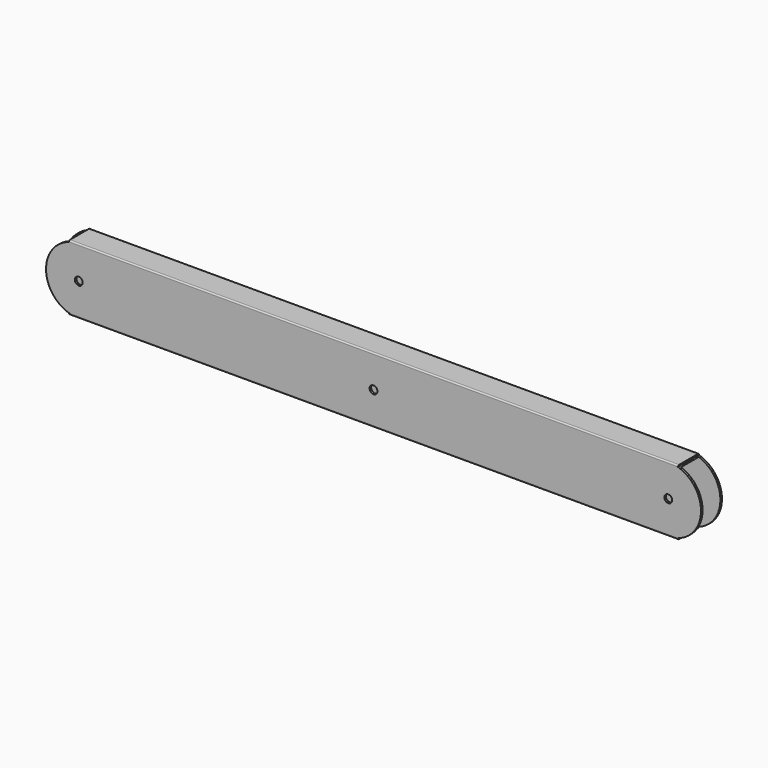
from build123d import *

# Parameters (mm, degrees)
F3_W     = 34
F3_H     = 94
F4_DEPTH = 500
F6_D     = 12
F6_DEPTH = 40
F6_TIP   = 3.6051637142
F7_DEPTH = 40
F8_DEPTH = 35
F9_DEPTH = 35


# Not quite as in the source:
# - a feature names something its author has since deleted; it is built from what else it names


with BuildPart() as f4:
    # F3 (on Right) → F4 (new body, symmetric)
    with BuildSketch(Plane.YZ):
        with BuildLine():
            ThreePointArc((-4.2945303673, -84.5), (-3.7087439297, -85.9142135624), (-2.2945303673, -86.5))
            Line((-2.2945303673, -86.5), (33.7054696327, -86.5))
            ThreePointArc((33.7054696327, -86.5), (35.1196831951, -85.9142135624), (35.7054696327, -84.5))
            Line((35.7054696327, -84.5), (35.7054696327, 11.5))
            ThreePointArc((35.7054696327, 11.5), (35.1196831951, 12.9142135624), (33.7054696327, 13.5))
            Line((33.7054696327, 13.5), (-2.2945303673, 13.5))
            ThreePointArc((-2.2945303673, 13.5), (-3.7087439297, 12.9142135624), (-4.2945303673, 11.5))
            Line((-4.2945303673, 11.5), (-4.2945303673, -84.5))
        make_face()
        with Locations((15.7054696327, -36.5)):
            Rectangle(F3_W, F3_H, mode=Mode.SUBTRACT)
    extrude(amount=F4_DEPTH, both=True)

    # F6
    with Locations(Plane.XZ.offset(4.2945303673)):
        with Locations((450, -36.2195856869), (0, -36.2195856869), (-450, -36.5)):
            Hole(F6_D / 2, depth=F6_DEPTH)
            with Locations((0, 0, -(F6_DEPTH + F6_TIP / 2))):  # 118° drill point
                Cone(0, F6_D / 2, F6_TIP, mode=Mode.SUBTRACT)

    # F5 (on face) → F7 (cut)
    with BuildSketch(Plane.XZ.offset(4.2945303673)):
        with BuildLine():
            ThreePointArc((-500, -36.5), (-490, -6.5), (-464, 11.5))
            Line((-464, 11.5), (-500, 11.5))
            Line((-500, 11.5), (-500, -36.5))
        make_face()
        with BuildLine():
            ThreePointArc((-464, -84.5), (-490, -66.5), (-500, -36.5))
            Line((-500, -36.5), (-500, -84.5))
            Line((-500, -84.5), (-464, -84.5))
        make_face()
        with BuildLine():
            Line((500, 11.5), (464, 11.5))
            ThreePointArc((464, 11.5), (490, -6.5), (500, -36.5))
            Line((500, -36.5), (500, 11.5))
        make_face()
        with BuildLine():
            Line((500, -84.5), (500, -36.5))
            ThreePointArc((500, -36.5), (490, -66.5), (464, -84.5))
            Line((464, -84.5), (500, -84.5))
        make_face()
    extrude(amount=-F7_DEPTH, mode=Mode.SUBTRACT)

    # F8 (cut): faces of the model
    f8_faces = [f4.faces().sort_by_distance(p)[0] for p in [
        (-500, 15.7054696327, 12.4878664624),
        (-500, 15.7054696327, -85.4878664624),
    ]]
    extrude(f8_faces, amount=-F8_DEPTH, mode=Mode.SUBTRACT)

    # F9 (cut): faces of the model
    f9_faces = [f4.faces().sort_by_distance(p)[0] for p in [
        (500, 15.7054696327, -85.4878664624),
        (500, 15.7054696327, 12.4878664624),
    ]]
    extrude(f9_faces, amount=-F9_DEPTH, mode=Mode.SUBTRACT)


solid = f4.part
